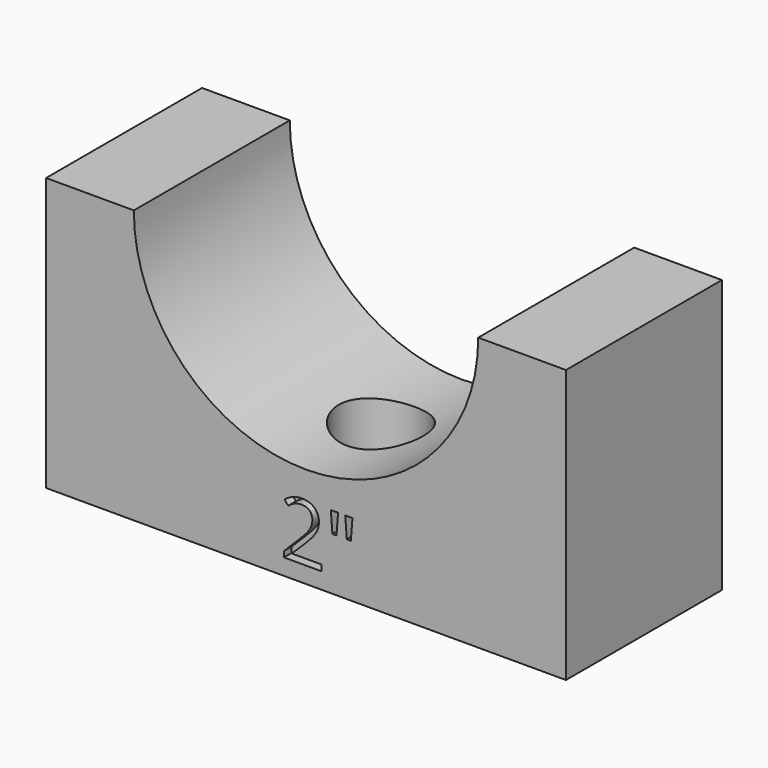
from build123d import *

# Parameters (mm, degrees)
F1_DEPTH       = 30
F3_D           = 9
F3_START       = 14.5000001
F3_CBORE_D     = 13
F3_CBORE_DEPTH = 9
F4_TEXT_SIZE   = 12.2780665859
F5_DEPTH       = 1.5


# Not quite as in the source:
# - Text() gives the source's letters only with a copy of the font that has no kerning and outlines rounded to 1/6400 em; it was checked with that copy


with BuildPart() as f1:
    # F0 (on Front) → F1 (new body)
    with BuildSketch(Plane.XZ):
        with BuildLine():
            Line((-40, -30), (40, -30))
            Line((40, -30), (40, 12))
            Line((40, 12), (26.5, 12))
            ThreePointArc((26.5, 12), (0, -14.5), (-26.5, 12))
            Line((-26.5, 12), (-40, 12))
            Line((-40, 12), (-40, -30))
        make_face()
    extrude(amount=F1_DEPTH)

    # F3 (through all)
    # its depths count from where the whole tool has entered the part; down to there all is cleared
    with Locations(Plane.XY.offset(-F3_START)):
        with Locations((0, -15.5798985064)):
            CounterBoreHole(F3_D / 2, F3_CBORE_D / 2, F3_CBORE_DEPTH)

    # F4 (on face) → F5 (cut)
    with BuildSketch(Plane.XZ.offset(30)):
        with Locations((-4, -27.5)):
            Text('2"', F4_TEXT_SIZE, font='Open Sans', text_align=(TextAlign.LEFT, TextAlign.BOTTOM))
    extrude(amount=-F5_DEPTH, mode=Mode.SUBTRACT)


solid = f1.part
